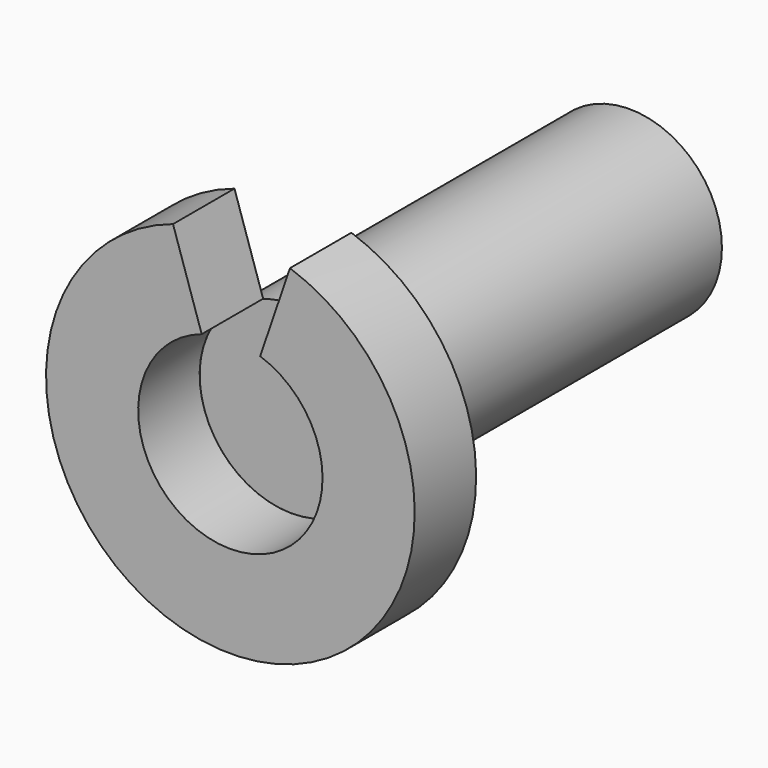
from build123d import *

# Parameters (mm, degrees)
F0_R     = 12
F1_DEPTH = 55
F2_R     = 24
F2_R_2   = 12
F3_DEPTH = 10
F5_DEPTH = 25


with BuildPart() as f1:
    # F0 (on Front) → F1 (new body)
    with BuildSketch(Plane.XZ):
        with Locations((-28.8248471916, 43.3525703847)):
            Circle(F0_R)
    extrude(amount=-F1_DEPTH)


with BuildPart() as f3:
    # F2 (on face) → F3 (new body)
    with BuildSketch(Plane.XZ):
        with Locations((-28.8248471916, 43.3525703847)):
            Circle(F2_R)
        with Locations((-28.8248471916, 43.3525703847)):
            Circle(F2_R_2, mode=Mode.SUBTRACT)
    extrude(amount=F3_DEPTH)

    # F4 (on face) → F5 (cut)
    with BuildSketch(Plane.XZ.offset(10)):
        with BuildLine():
            Line((-36.2911306636, 66.1616609215), (-32.5579889276, 54.7571156531))
            ThreePointArc((-32.5579889276, 54.7571156531), (-28.7472060364, 55.3523192092), (-24.9444440878, 54.707854254))
            Line((-24.9444440878, 54.707854254), (-21.0640409839, 66.0631381233))
            ThreePointArc((-21.0640409839, 66.0631381233), (-28.6695648813, 67.3520680337), (-36.2911306636, 66.1616609215))
        make_face()
    extrude(amount=-F5_DEPTH, mode=Mode.SUBTRACT)


solid = Compound([f1.part, f3.part])
